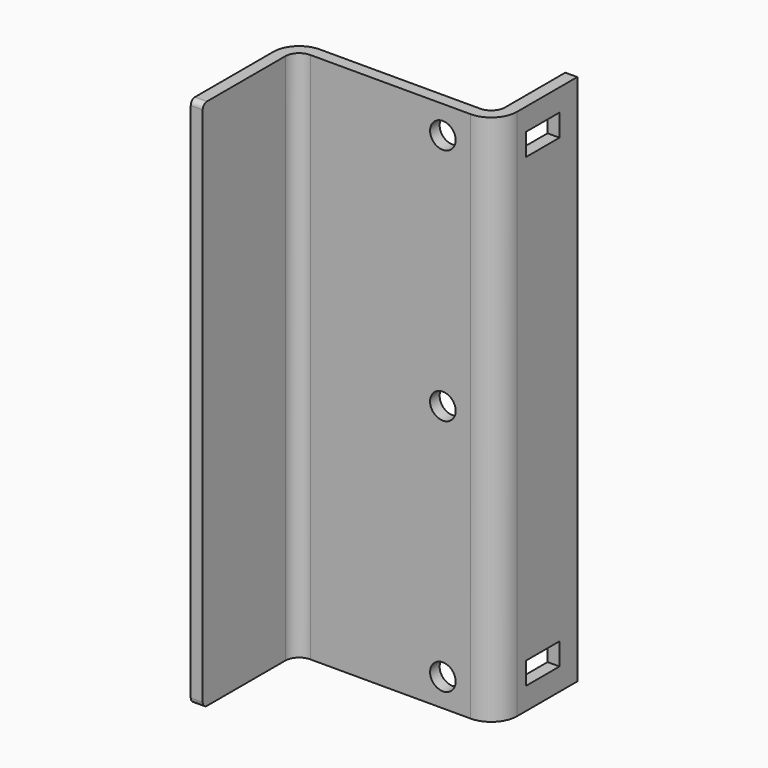
from build123d import *

# Parameters (mm, degrees)
F1_DEPTH = 76.1175008
F2_R     = 1.98374
F3_R     = 3.69316
F4_R     = 1.8288
F5_DEPTH = 1.70942
F6_R     = 0.762
F7_W     = 6
F7_H     = 3.175
F8_DEPTH = 1.70942


# Not quite as in the source:
# - a feature names something its author has since deleted; it is built from what else it names


with BuildPart() as f1:
    # F0 (on Top) → F1 (new body)
    with BuildSketch(Plane.XY):
        Polygon((-1.70942, 0), (0, 0), (0, 16.7533828), (28.6143954, 16.7533828), (28.6143954, 31.2090308), (26.9049754, 31.2090308), (26.9049754, 18.4628028), (-1.70942, 18.4628028), align=None)
    extrude(amount=F1_DEPTH)

    # F2
    f2_edges = [f1.edges().sort_by_distance(p)[0] for p in [
        (0, 16.753383, 38.05875),
        (26.904975, 18.462803, 38.05875),
    ]]
    fillet(f2_edges, radius=F2_R)

    # F3
    f3_edges = [f1.edges().sort_by_distance(p)[0] for p in [
        (-1.70942, 18.462803, 38.05875),
        (28.614395, 16.753383, 38.05875),
    ]]
    fillet(f3_edges, radius=F3_R)

    # F4 (on face) → F5 (cut, through all)
    with BuildSketch(Plane.XZ.offset(-16.7533828)):
        with Locations((20.9524854, 72.1487508)):
            Circle(F4_R)
        with Locations((20.9524854, 38.0587504)):
            Circle(F4_R)
        with Locations((20.9524854, 3.96875)):
            Circle(F4_R)
    extrude(amount=-F5_DEPTH, mode=Mode.SUBTRACT)

    # F6
    f6_edges = [f1.edges().sort_by_distance(p)[0] for p in [
        (-0.85471, 0, 76.117501),
        (-0.85471, 0, 0),
    ]]
    fillet(f6_edges, radius=F6_R)

    # F7 (on face) → F8 (cut, through all)
    with BuildSketch(Plane(origin=(26.9049754, 0, 0), x_dir=(0, -1, 0), z_dir=(-1, 0, 0))):
        with Locations((-25.0340308, 71.3550008)):
            Rectangle(F7_W, F7_H)
        with Locations((-25.0340308, 4.7625)):
            Rectangle(F7_W, F7_H)
    extrude(amount=-F8_DEPTH, mode=Mode.SUBTRACT)


solid = f1.part
